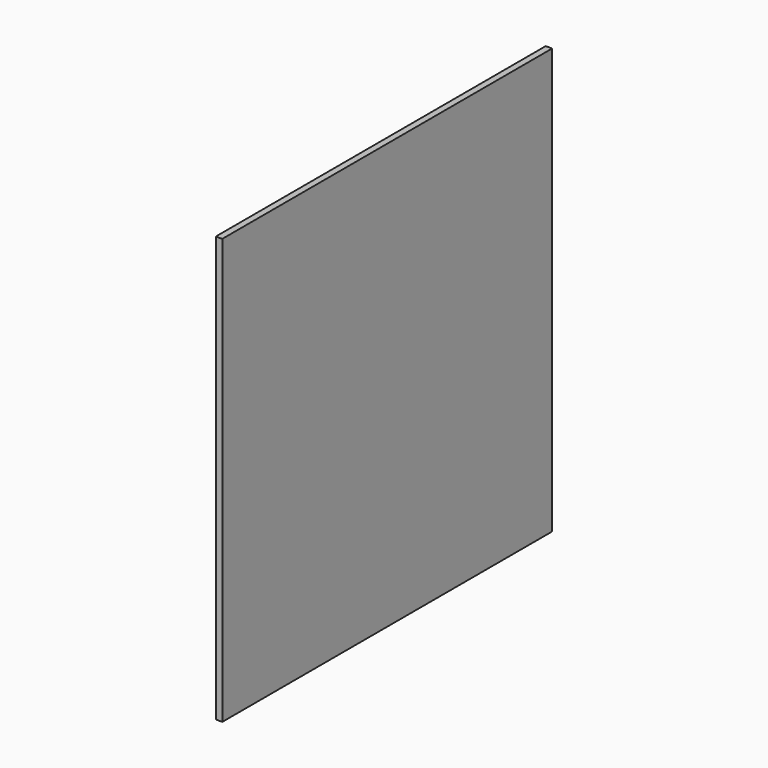
from build123d import *

# Parameters (mm, degrees)
F0_W     = 812.8
F0_H     = 838.2
F1_DEPTH = 12.7


# Not quite as in the source:
# - a length typed as a fraction of an inch, garbled in the dataset ("3 / 203.2 mm" for 3/8 in), is restored


with BuildPart() as f1:
    # F0 (on Right) → F1 (new body)
    with BuildSketch(Plane.YZ):
        with Locations((6.9073382765, 41.1031354467)):
            Rectangle(F0_W, F0_H)
    extrude(amount=F1_DEPTH)


solid = f1.part
